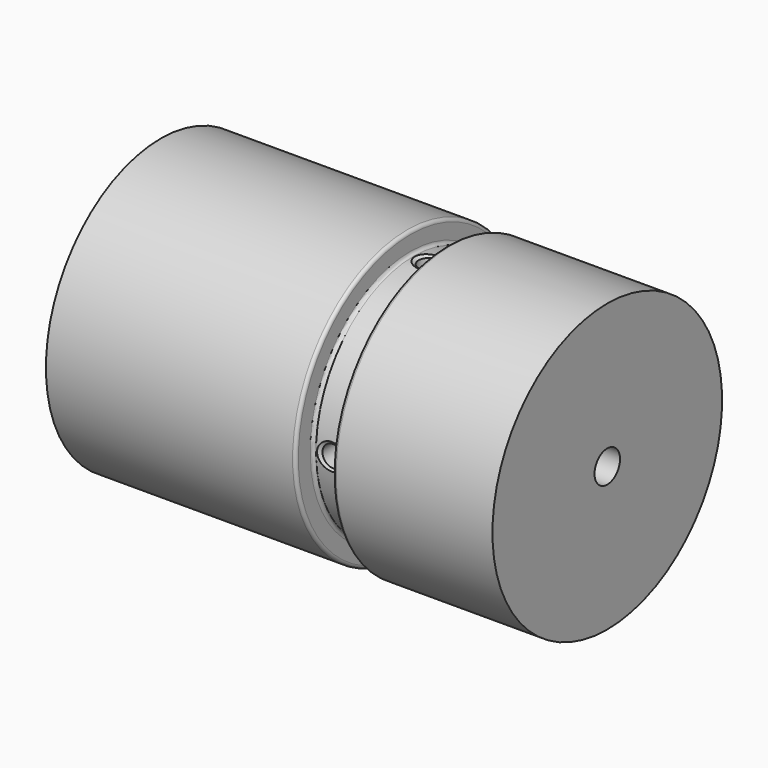
from build123d import *

# Parameters (mm, degrees)
F0_W            = 42
F0_H            = 12
F2_W            = 3.5
F2_H            = 2
F4_R            = 0.3
F6_COPIES_COUNT = 4


# Not quite as in the source:
# - a pattern or mirror of a feature is missing from the dataset's text; its kind, count and spacing are read off the source's solid


with BuildPart() as f1:
    # F0 (on Front) → F1 (revolve)
    with BuildSketch(Plane.XZ):
        with Locations((-21, 7.5)):
            Rectangle(F0_W, F0_H)
    revolve(axis=Axis((-10.2689703926, 0, 0), (1, 0, 0)))

    # F2 (on face) → F3 (revolve, cut)
    with BuildSketch(Plane.XZ):
        with Locations((-16.75, 12.5)):
            Rectangle(F2_W, F2_H)
    revolve(axis=Axis((-21, 0, 0), (-1, 0, 0)), mode=Mode.SUBTRACT)

    # F4
    f4_edges = [f1.edges().sort_by_distance(p)[0] for p in [
        (-18.5, 0, -13.5),
        (-15, 0, -13.5),
        (-18.5, 0, -11.5),
        (-15, 0, -11.5),
    ]]
    fillet(f4_edges, radius=F4_R)

    # F5 (on face) → F6 (revolve, cut)
    with BuildSketch(Plane.XZ):
        Polygon((-15.4035898385, 11.5), (-16.75, 11.5), (-16.75, 0), (-15.75, 0), (-15.75, 11.3), align=None)
    f6 = revolve(axis=Axis((-16.75, 0, 5.75), (0, 0, 1)), mode=Mode.SUBTRACT)

    # F6_copies: F6 ×4 about axis
    f6_copies_axis = Axis((0, 0, 0), (1, 0, 0))
    for i in range(1, F6_COPIES_COUNT):
        add(f6.rotate(f6_copies_axis, i * 360 / F6_COPIES_COUNT), mode=Mode.SUBTRACT)


solid = f1.part
